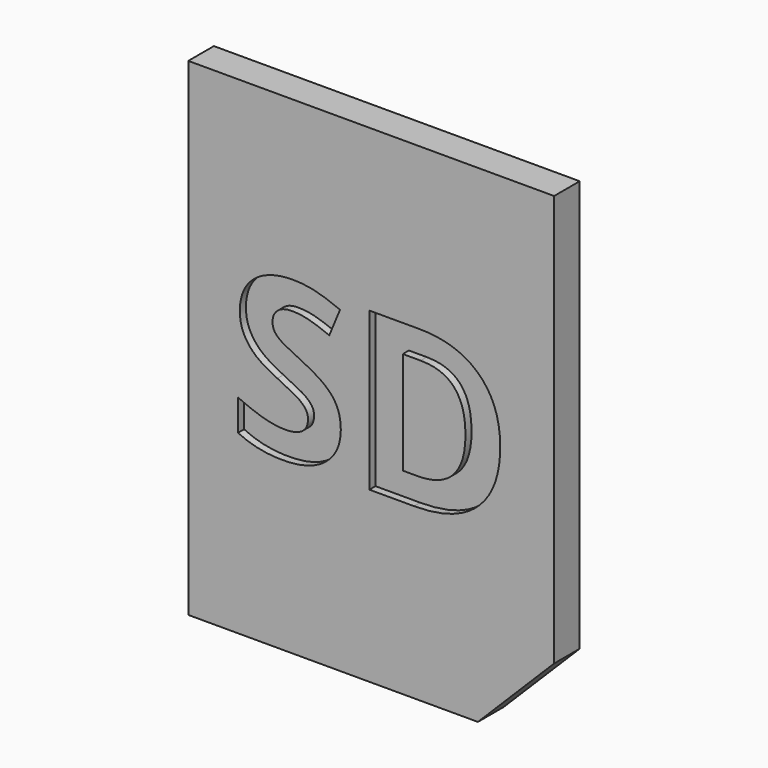
from build123d import *

# Parameters (mm, degrees)
F0_W         = 24
F0_H         = 32
F1_DEPTH     = 2.1
F2_SIZE      = 5
F3_TEXT_SIZE = 14.490430667
F4_DEPTH     = 0.5


# Not quite as in the source:
# - Text() gives the source's letters only with a copy of the font that has no kerning and outlines rounded to 1/6400 em; it was checked with that copy


with BuildPart() as f1:
    # F0 (on Front) → F1 (new body)
    with BuildSketch(Plane.XZ):
        Rectangle(F0_W, F0_H)
    extrude(amount=F1_DEPTH)

    # F2
    f2_edges = [f1.edges().sort_by_distance(p)[0] for p in [
        (12, -1.05, -16),
    ]]
    chamfer(f2_edges, length=F2_SIZE)

    # F3 (on face) → F4 (cut)
    with BuildSketch(Plane.XZ.offset(2.1)):
        with Locations((-9.402931025, -4.9011731829)):
            Text('SD', F3_TEXT_SIZE, font='Open Sans', font_style=FontStyle.BOLD, text_align=(TextAlign.LEFT, TextAlign.BOTTOM))
    extrude(amount=-F4_DEPTH, mode=Mode.SUBTRACT)


solid = f1.part
